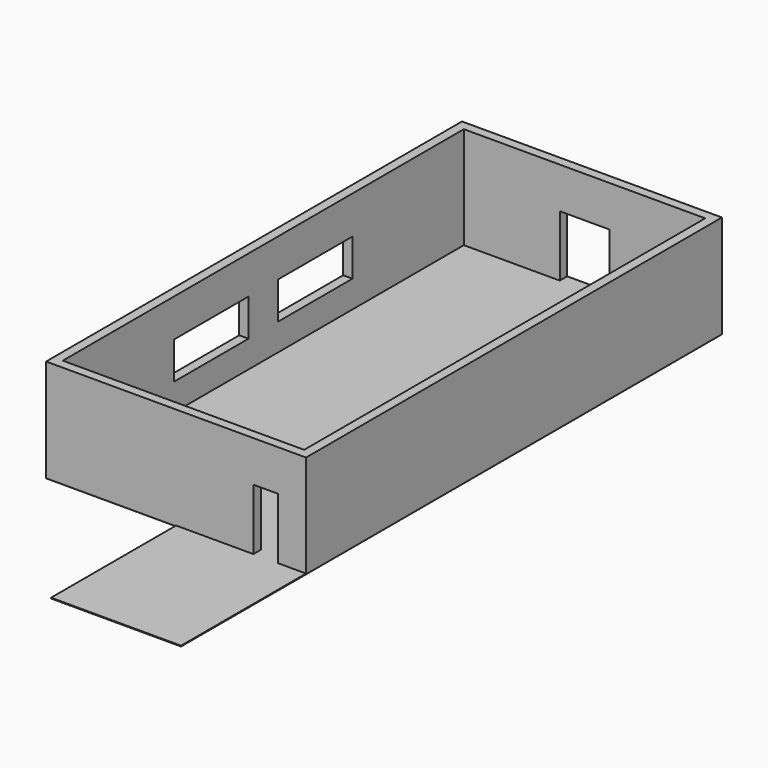
from build123d import *

# Parameters (mm, degrees)
F0_W     = 8534.4
F0_H     = 17068.8
F0_W_2   = 7924.8
F0_H_2   = 16459.2
F1_DEPTH = 3352.8
F3_DEPTH = 25.4
F4_W     = 812.8
F4_H     = 2032
F5_DEPTH = 304.8
F6_W     = 3048
F6_H     = 1219.2
F7_DEPTH = 304.8
F9_DEPTH = 304.8


with BuildPart() as f1:
    # F0 (on Top) → F1 (new body)
    with BuildSketch(Plane.XY):
        Rectangle(F0_W, F0_H)
        Rectangle(F0_W_2, F0_H_2, mode=Mode.SUBTRACT)
    extrude(amount=F1_DEPTH)

    # F4 (on face) → F5 (cut, through all)
    with BuildSketch(Plane.XZ.offset(8534.4)):
        with Locations((2946.4, 990.6)):
            Rectangle(F4_W, F4_H)
    extrude(amount=-F5_DEPTH, mode=Mode.SUBTRACT)

    # F6 (on face) → F7 (cut, through all)
    with BuildSketch(Plane(origin=(-4267.2, 0, 0), x_dir=(0, -1, 0), z_dir=(-1, 0, 0))):
        with Locations((-2133.6, 1498.6)):
            Rectangle(F6_W, F6_H)
        with Locations((2133.6, 1498.6)):
            Rectangle(F6_W, F6_H)
    extrude(amount=-F7_DEPTH, mode=Mode.SUBTRACT)

    # F8 (on face) → F9 (cut, through all)
    with BuildSketch(Plane(origin=(0, 8534.4, 0), x_dir=(-1, 0, 0), z_dir=(0, 1, 0))):
        Polygon((812.8, 2006.6), (0, 2006.6), (-812.8, 2006.6), (-812.8, -25.4), (0, -25.4), (812.8, -25.4), align=None)
    extrude(amount=-F9_DEPTH, mode=Mode.SUBTRACT)


with BuildPart() as f3:
    # F2 (on face) → F3 (new body)
    with BuildSketch(Plane(origin=(0, 0, 0), x_dir=(1, 0, 0), z_dir=(0, 0, -1))):
        Polygon((0, 8534.4), (-4267.2, 8534.4), (-4267.2, -8534.4), (4267.2, -8534.4), (4267.2, 8534.4), (4267.2, 13663.9823913574), (0, 13663.9823913574), align=None)
    extrude(amount=F3_DEPTH)


solid = Compound([f1.part, f3.part])
